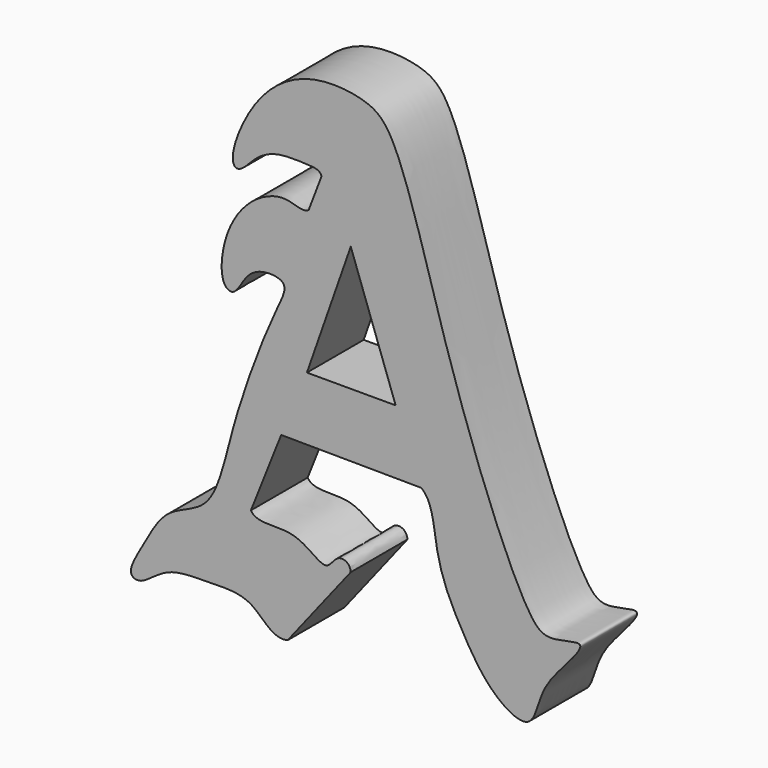
from build123d import *

# Parameters (mm, degrees)
F2_DEPTH = 6.35


with BuildPart() as f2:
    # F0 (on Front) → F2 (new body)
    with BuildSketch(Plane.XZ):
        with BuildLine():
            add(Edge.make_bspline(
                [(-5.6547205895, -14.3365655094), (-7.0301308965, -14.6692847815), (-8.63646893, -11.8338371449), (-12.6586229193, -12.1363609257), (-16.5427947807, -11.9703002383), (-18.6312785028, -14.2459332261), (-20.1753261579, -13.691267767), (-18.3817454418, -10.7549540998), (-16.5880310826, -7.2693282581), (-12.090098104, -6.5155976165), (-10.7268601383, 1.3284755436), (-7.15035983, 10.6370147616), (-5.3111997393, 13.9329612279), (-8.0493431527, 14.1823809395), (-9.5051874807, 13.1525759378), (-10.3539445589, 11.2015570355), (-11.7933586196, 11.8843985956), (-11.4315691698, 16.2189016599), (-8.8371104329, 19.7062529683), (-5.7177325321, 20.7532793843), (-4.3266438554, 19.8177589978), (-3.7674787454, 20.1842412353)],
                knots=[0, 0, 0, 0, 0.0203892715, 0.0412074472, 0.0622089842, 0.0798889909, 0.0896985978, 0.1078237394, 0.129128868, 0.149432843, 0.1785546542, 0.2134586028, 0.2306922687, 0.245134567, 0.259733303, 0.2740070502, 0.2840016317, 0.3051566024, 0.3276468472, 0.3459860162, 0.3606548005, 0.3606548005, 0.3606548005, 0.3606548005], degree=3))
            Line((-5.6547205895, -14.3365655094), (0, -7.1329348721))
            add(Edge.make_bspline(
                [(-8.9392503724, -5.1691527478), (-8.3654029688, -6.1027103997), (-4.8800205477, -4.9944999403), (-2.1681694978, -8.2238494187), (-1.2903858198, -5.9460625327), (-0.0570759533, -6.4478163395), (0, -7.1329348721)],
                knots=[0.9024298628, 0.9024298628, 0.9024298628, 0.9024298628, 0.9234974476, 0.9426262213, 0.9555091115, 0.9677426818, 0.9677426818, 0.9677426818, 0.9677426818], degree=3))
            add(Edge.make_bspline(
                [(-6.2273619696, 1.6573261237), (-8.1571238525, 0.2387861816), (-9.7261491674, -3.8889946661), (-8.9392503724, -5.1691527478)],
                knots=[0.87354055, 0.87354055, 0.87354055, 0.87354055, 0.9024298628, 0.9024298628, 0.9024298628, 0.9024298628], degree=3))
            add(Edge.make_bspline(
                [(6.3034351915, 1.5638129553), (5.0512890113, 2.4614749756), (-0.270467213, 0.974484873), (-4.450124604, 2.9637475076), (-6.2273619696, 1.6573261237)],
                knots=[0.820159406, 0.820159406, 0.820159406, 0.820159406, 0.8469345906, 0.87354055, 0.87354055, 0.87354055, 0.87354055], degree=3))
            add(Edge.make_bspline(
                [(-2.6172876824, 23.2060495764), (-2.7504274329, 23.6673500074), (-3.9273703778, 23.732459794), (-6.7993760502, 23.8905815965), (-8.645232641, 22.6948188039), (-9.5507095241, 21.5518513633), (-10.3490816321, 21.2238199588), (-10.8767561118, 22.4214945327), (-8.7142751374, 27.774908602), (-4.0784113472, 31.0949001576), (1.1902189676, 30.6940663093), (4.4376310941, 28.668622615), (8.492288771, 11.9474647708), (15.292983919, -5.1047749298), (17.6830588612, -6.912726707), (21.7499000452, -5.3967962413), (18.4975174925, -8.9398570877), (16.9444889997, -10.9768788506), (16.2612606887, -14.7008093867), (12.4974303238, -12.6818460945), (9.9347955146, -8.6054380584), (7.4008489181, -3.6127481897), (7.4178992577, 0.7648550692), (6.3034351915, 1.5638129553)],
                knots=[0.3798217217, 0.3798217217, 0.3798217217, 0.3798217217, 0.3919575446, 0.4102153796, 0.4258781621, 0.4386849161, 0.4470921999, 0.4568264408, 0.4817171565, 0.5072690713, 0.530502364, 0.5492559702, 0.5937441178, 0.6396917328, 0.6563370883, 0.6730129651, 0.6913431153, 0.710536078, 0.7281104592, 0.7466389971, 0.7705033569, 0.7963283378, 0.820159406, 0.820159406, 0.820159406, 0.820159406], degree=3))
            add(Edge.make_bspline(
                [(-3.7674787454, 20.1842412353), (-3.0368474003, 20.6631041066), (-2.4070111209, 22.4774867838), (-2.6172876824, 23.2060495764)],
                knots=[0.3606548005, 0.3606548005, 0.3606548005, 0.3606548005, 0.3798217217, 0.3798217217, 0.3798217217, 0.3798217217], degree=3))
        make_face()
        Polygon((-3.9230575785, 7.3187039234), (0, 18.5261722654), (4.0186583064, 7.3187039234), align=None, mode=Mode.SUBTRACT)
        with BuildLine():
            Line((-2.6172876824, 23.2060495764), (-3.7674787454, 20.1842412353))
            add(Edge.make_bspline(
                [(-3.7674787454, 20.1842412353), (-3.0368474003, 20.6631041066), (-2.4070111209, 22.4774867838), (-2.6172876824, 23.2060495764)],
                knots=[0.3606548005, 0.3606548005, 0.3606548005, 0.3606548005, 0.3798217217, 0.3798217217, 0.3798217217, 0.3798217217], degree=3))
        make_face()
        with BuildLine():
            add(Edge.make_bspline(
                [(-6.2273619696, 1.6573261237), (-8.1571238525, 0.2387861816), (-9.7261491674, -3.8889946661), (-8.9392503724, -5.1691527478)],
                knots=[0.87354055, 0.87354055, 0.87354055, 0.87354055, 0.9024298628, 0.9024298628, 0.9024298628, 0.9024298628], degree=3))
            Line((-8.9392503724, -5.1691527478), (-6.2273619696, 1.6573261237))
        make_face()
        with BuildLine():
            Line((-6.2273619696, 1.6573261237), (6.3034351915, 1.5638129553))
            add(Edge.make_bspline(
                [(6.3034351915, 1.5638129553), (5.0512890113, 2.4614749756), (-0.270467213, 0.974484873), (-4.450124604, 2.9637475076), (-6.2273619696, 1.6573261237)],
                knots=[0.820159406, 0.820159406, 0.820159406, 0.820159406, 0.8469345906, 0.87354055, 0.87354055, 0.87354055, 0.87354055], degree=3))
        make_face()
    extrude(amount=F2_DEPTH)


solid = f2.part
